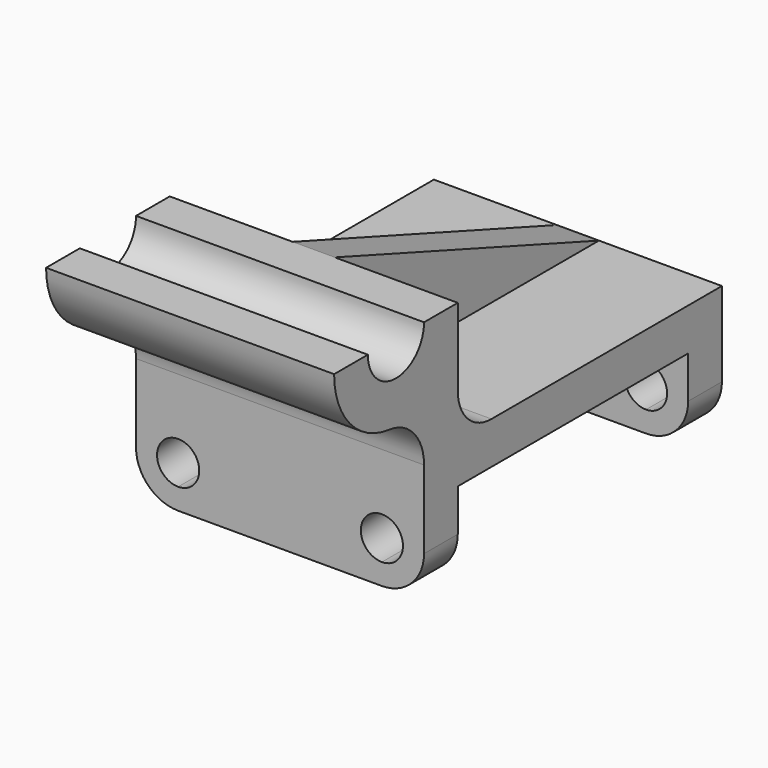
from build123d import *

# Parameters (mm, degrees)
F0_W      = 82
F0_H      = 106
F1_DEPTH  = 36
F3_R      = 12
F4_DEPTH  = 191.1
F5_R      = 12
F7_DEPTH  = 174.6
F9_W      = 82
F9_H      = 12.96312543
F10_DEPTH = 116.9
F12_DEPTH = 34
F14_DEPTH = 25
F15_W     = 12
F15_H     = 34
F16_DEPTH = 25
F18_DEPTH = 34
F19_R     = 12
F21_DEPTH = 82
F22_R     = 14


# Not quite as in the source:
# - a feature of the source that left no trace in its solid (it failed there, or was rolled back) is left out


with BuildPart() as f1:
    # F0 (on Top) → F1 (new body)
    with BuildSketch(Plane.XY):
        Rectangle(F0_W, F0_H)
    extrude(amount=F1_DEPTH)

    # F3
    f3_edges = [f1.edges().sort_by_distance(p)[0] for p in [
        (-41, 0, 0),
    ]]
    fillet(f3_edges, radius=F3_R)

    # F2 (on face) → F4 (cut)
    with BuildSketch(Plane.XZ.offset(53)):
        with BuildLine():
            ThreePointArc((-29, 18), (-35, 12), (-29, 6))
            Line((-29, 6), (-29, 12))
            Line((-29, 12), (-29, 18))
        make_face()
        with BuildLine():
            Line((-29, 12), (-29, 6))
            ThreePointArc((-29, 6), (-24.7573593129, 7.7573593129), (-23, 12))
            ThreePointArc((-23, 12), (-24.7573593129, 16.2426406871), (-29, 18))
            Line((-29, 18), (-29, 12))
        make_face()
        with BuildLine():
            Line((29, 12), (29, 6))
            ThreePointArc((29, 6), (33.2426406871, 7.7573593129), (35, 12))
            ThreePointArc((35, 12), (33.2426406871, 16.2426406871), (29, 18))
            Line((29, 18), (29, 12))
        make_face()
        with BuildLine():
            ThreePointArc((29, 18), (23, 12), (29, 6))
            Line((29, 6), (29, 12))
            Line((29, 12), (29, 18))
        make_face()
    extrude(amount=-F4_DEPTH, mode=Mode.SUBTRACT)

    # F5
    f5_edges = [f1.edges().sort_by_distance(p)[0] for p in [
        (41, 0, 0),
    ]]
    fillet(f5_edges, radius=F5_R)

    # F6 (on face) → F7 (cut)
    with BuildSketch(Plane.YZ.offset(41)):
        Polygon((41, 24), (-30.1027745008, 24), (-41, 24), (-41, 12), (41, 12), align=None)
    extrude(amount=-F7_DEPTH, mode=Mode.SUBTRACT)

    # F9 (on face) → F10 (cut)
    with BuildSketch(Plane.YZ.offset(41)):
        with Locations((0, 5.518437285)):
            Rectangle(F9_W, F9_H)
    extrude(amount=-F10_DEPTH, mode=Mode.SUBTRACT)

    # F11 (on face) → F12 (join)
    with BuildSketch(Plane.XY.offset(36)):
        Polygon((0, 53), (-6, 53), (-6, -53), (6, -53), (6, 53), align=None)
    extrude(amount=F12_DEPTH)

    # F13 (on face) → F14 (cut)
    with BuildSketch(Plane(origin=(-6, 0, 0), x_dir=(0, -1, 0), z_dir=(-1, 0, 0))):
        Polygon((-53, 70), (-53, 36), (41, 70), align=None)
    extrude(amount=-F14_DEPTH, mode=Mode.SUBTRACT)

    # F15 (on face) → F16 (cut)
    with BuildSketch(Plane(origin=(-6, 0, 0), x_dir=(0, -1, 0), z_dir=(-1, 0, 0))):
        with Locations((47, 53)):
            Rectangle(F15_W, F15_H)
    extrude(amount=-F16_DEPTH, mode=Mode.SUBTRACT)

    # F17 (on face) → F18 (join)
    with BuildSketch(Plane.XY.offset(36)):
        Polygon((41, -53), (41, -41), (6, -41), (-6, -41), (-41, -41), (-41, -53), align=None)
    extrude(amount=F18_DEPTH)

    # F19
    f19_edges = [f1.edges().sort_by_distance(p)[0] for p in [
        (-23.5, -41, 36),
        (23.5, -41, 36),
    ]]
    fillet(f19_edges, radius=F19_R)

    # F20 (on face) → F21 (join, through all)
    with BuildSketch(Plane(origin=(-41, 0, 0), x_dir=(0, -1, 0), z_dir=(-1, 0, 0))):
        with BuildLine():
            Line((53, 70), (53, 50.4040820577))
            ThreePointArc((53, 50.4040820577), (74.4891252931, 51.2383369607), (85, 70))
            Line((85, 70), (73, 70))
            ThreePointArc((73, 70), (63, 60), (53, 70))
        make_face()
        with BuildLine():
            Line((53, 70), (41, 70))
            ThreePointArc((41, 70), (44.2383369607, 58.5108747069), (53, 50.4040820577))
            Line((53, 50.4040820577), (53, 70))
        make_face()
    extrude(amount=-F21_DEPTH)

    # F22
    f22_edges = [f1.edges().sort_by_distance(p)[0] for p in [
        (0, -53, 50.404082),
    ]]
    fillet(f22_edges, radius=F22_R)


solid = f1.part
